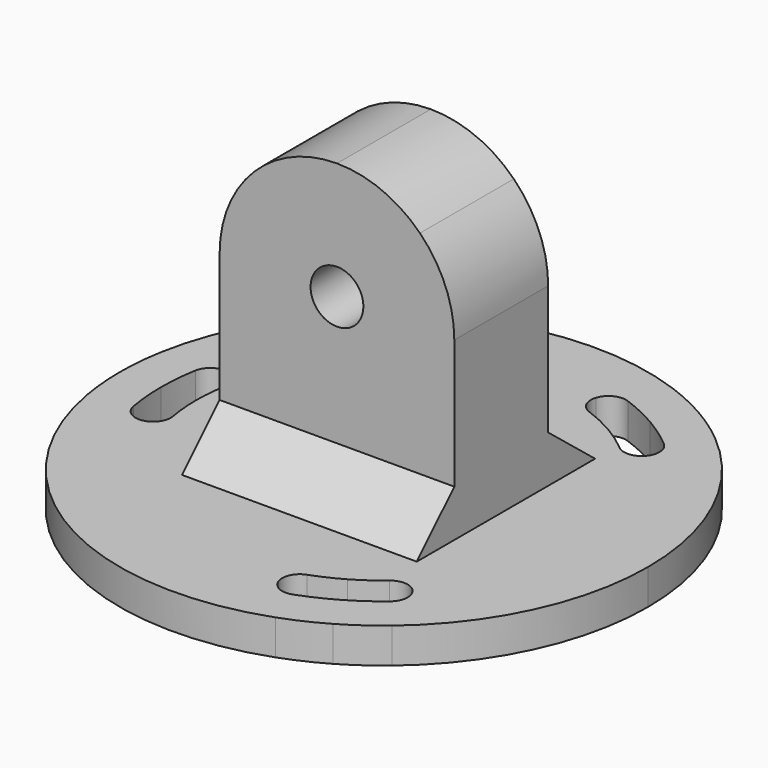
from build123d import *

# Parameters (mm, degrees)
F1_DEPTH = 6
F2_W     = 40
F2_H     = 20
F3_DEPTH = 50
F5_DEPTH = 40
F7_DEPTH = 30
F8_DEPTH = 30


# Not quite as in the source:
# - ends of sketch curves that miss each other by under 0.0002 mm in the source are joined


with BuildPart() as f1:
    # F0 (on Top) → F1 (new body)
    with BuildSketch(Plane.XY):
        with BuildLine():
            ThreePointArc((28.9254424359, -34.4719999404), (40.7838504166, -19.0178217783), (45, 0))
            ThreePointArc((45, 0), (40.7838504166, 19.0178217783), (28.9254424359, 34.4719999404))
            Line((28.9254424359, 34.4719999404), (24.4259291681, 29.1096888385))
            ThreePointArc((24.4259292345, 29.1096887828), (34.4396959257, 16.0594939069), (38, 0))
            ThreePointArc((38, 0), (34.4396959, -16.059493962), (24.4259291412, -29.1096888611))
            Line((24.4259291681, -29.1096888385), (28.9254424359, -34.4719999404))
        make_face()
        with BuildLine():
            ThreePointArc((22.5, -38.9711431703), (25.8109396358, -36.861841993), (28.9254424359, -34.4719999404))
            Line((28.9254424359, -34.4719999404), (24.4259291681, -29.1096888385))
            ThreePointArc((24.4259291412, -29.1096888611), (21.795904567, -31.127777693), (19, -32.9089653438))
            Line((19, -32.9089653438), (22.5, -38.9711431703))
        make_face()
        with BuildLine():
            ThreePointArc((15.3909064497, -42.2861679354), (19.0178217783, -40.7838504166), (22.5, -38.9711431703))
            Line((22.5, -38.9711431703), (19, -32.9089653438))
            ThreePointArc((19, -32.9089653438), (16.0594939837, -34.4396958899), (12.9967655243, -35.7083195615))
            Line((12.9967654464, -35.7083195899), (15.3909064497, -42.2861679354))
        make_face()
        with BuildLine():
            ThreePointArc((-44.3163488855, -7.814167995), (-22.5, -38.9711431703), (15.3909064497, -42.2861679354))
            Line((15.3909064497, -42.2861679354), (12.9967654464, -35.7083195899))
            ThreePointArc((12.9967655243, -35.7083195615), (-18.9999999457, -32.9089653752), (-37.4226946071, -6.5986307931))
            Line((-37.4226946145, -6.5986307513), (-44.3163488855, -7.814167995))
        make_face()
        with BuildLine():
            ThreePointArc((-37.4226946071, -6.5986307931), (-18.9999999457, -32.9089653752), (12.9967655243, -35.7083195615))
            ThreePointArc((12.9967655243, -35.7083195615), (10.6448654939, -35.5803659462), (9.1102432746, -33.7935418013))
            ThreePointArc((9.1102432746, -33.7935418013), (-17.5, -30.3108891325), (-33.8211873211, -9.0070687902))
            ThreePointArc((-33.8211873211, -9.0070687902), (-36.1359334802, -8.5714590704), (-37.4226946071, -6.5986307931))
        make_face()
        with BuildLine():
            ThreePointArc((-33.8211873211, -9.0070687902), (-17.5, -30.3108891325), (9.1102432746, -33.7935418013))
            ThreePointArc((9.1102432746, -33.7935418013), (9.2795808611, -31.5634020763), (10.9446447781, -30.0701637954))
            ThreePointArc((10.9446447781, -30.0701637954), (-15.9999999119, -27.712812972), (-31.5138480965, -5.5567416849))
            ThreePointArc((-31.5138480965, -5.5567416849), (-31.4796872612, -5.8162189899), (-31.4682713554, -6.0776862183))
            ThreePointArc((-31.4682713554, -6.0776862183), (-32.1293344064, -7.956349027), (-33.8211873211, -9.0070687902))
        make_face()
        with BuildLine():
            Line((10.9446445864, -30.0701638651), (0, 0))
            Line((0, 0), (-31.5138480964, -5.5567416853))
            ThreePointArc((-31.5138480964, -5.5567416853), (-15.9999999119, -27.712812972), (10.9446445864, -30.0701638651))
        make_face()
        with BuildLine():
            Line((-31.5138480964, -5.5567416853), (0, 0))
            Line((0, 0), (-32, 0))
            ThreePointArc((-32, 0), (-31.878230339, -2.7889837677), (-31.5138480965, -5.5567416849))
        make_face()
        with BuildLine():
            Line((-32, 0), (0, 0))
            Line((0, 0), (-31.5138480964, 5.5567416853))
            ThreePointArc((-31.5138480966, 5.5567416843), (-31.878230339, 2.7889837674), (-32, 0))
        make_face()
        with BuildLine():
            ThreePointArc((-45, 0), (-44.8287614141, -3.9220084236), (-44.3163488855, -7.814167995))
            Line((-44.3163488855, -7.814167995), (-37.4226946145, -6.5986307513))
            ThreePointArc((-37.4226946071, -6.5986307931), (-37.8553985256, -3.3119182456), (-38, 0))
            Line((-38, 0), (-45, 0))
        make_face()
        with BuildLine():
            Line((-37.4226946145, 6.5986307513), (-44.3163488855, 7.814167995))
            ThreePointArc((-44.3163488855, 7.814167995), (-44.8287614141, 3.9220084236), (-45, 0))
            Line((-45, 0), (-38, 0))
            ThreePointArc((-38, 0), (-37.8553985261, 3.3119182405), (-37.4226946089, 6.5986307831))
        make_face()
        with BuildLine():
            Line((12.9967654464, 35.7083195899), (15.3909064497, 42.2861679354))
            ThreePointArc((15.3909064497, 42.2861679354), (-22.5, 38.9711431703), (-44.3163488855, 7.814167995))
            Line((-44.3163488855, 7.814167995), (-37.4226946145, 6.5986307513))
            ThreePointArc((-37.4226946089, 6.5986307831), (-18.9999999501, 32.9089653726), (12.9967655243, 35.7083195615))
        make_face()
        with BuildLine():
            ThreePointArc((9.1102432746, 33.7935418013), (10.6448654939, 35.5803659462), (12.9967655243, 35.7083195615))
            ThreePointArc((12.9967655243, 35.7083195615), (-18.9999999501, 32.9089653726), (-37.4226946089, 6.5986307831))
            ThreePointArc((-37.4226946089, 6.5986307831), (-36.1359334844, 8.5714590676), (-33.8211873211, 9.0070687902))
            ThreePointArc((-33.8211873211, 9.0070687902), (-17.5, 30.3108891325), (9.1102432746, 33.7935418013))
        make_face()
        with BuildLine():
            Line((-31.5138480964, 5.5567416853), (0, 0))
            Line((0, 0), (10.9446445864, 30.0701638651))
            ThreePointArc((10.9446445864, 30.0701638651), (-15.9999999047, 27.7128129761), (-31.5138480964, 5.5567416853))
        make_face()
        with BuildLine():
            ThreePointArc((10.9446447943, 30.0701637895), (9.2795808649, 31.5634020686), (9.1102432746, 33.7935418013))
            ThreePointArc((9.1102432746, 33.7935418013), (-17.5, 30.3108891325), (-33.8211873211, 9.0070687902))
            ThreePointArc((-33.8211873211, 9.0070687902), (-32.1293344064, 7.956349027), (-31.4682713554, 6.0776862183))
            ThreePointArc((-31.4682713554, 6.0776862183), (-31.4796872612, 5.8162189895), (-31.5138480966, 5.5567416843))
            ThreePointArc((-31.5138480966, 5.5567416843), (-15.9999999047, 27.7128129761), (10.9446447943, 30.0701637895))
        make_face()
        with BuildLine():
            Line((19, 32.9089653438), (22.5, 38.9711431703))
            ThreePointArc((22.5, 38.9711431703), (19.0178217783, 40.7838504166), (15.3909064497, 42.2861679354))
            Line((15.3909064497, 42.2861679354), (12.9967654464, 35.7083195899))
            ThreePointArc((12.9967655243, 35.7083195615), (16.0594939837, 34.4396958899), (19, 32.9089653438))
        make_face()
        with BuildLine():
            Line((24.4259291681, 29.1096888385), (28.9254424359, 34.4719999404))
            ThreePointArc((28.9254424359, 34.4719999404), (25.8109396358, 36.861841993), (22.5, 38.9711431703))
            Line((22.5, 38.9711431703), (19, 32.9089653438))
            ThreePointArc((19, 32.9089653438), (21.7959046168, 31.1277776581), (24.4259292345, 29.1096887828))
        make_face()
        with BuildLine():
            Line((0, 0), (20.56920351, 24.5134221798))
            ThreePointArc((20.5692034907, 24.5134221959), (18.354445953, 26.2128654244), (16, 27.7128129211))
            Line((16, 27.7128129211), (0, 0))
        make_face()
        with BuildLine():
            Line((0, 0), (16, 27.7128129211))
            ThreePointArc((16, 27.7128129211), (13.523784476, 29.0018491384), (10.9446447943, 30.0701637895))
            Line((10.9446447943, 30.0701637895), (0, 0))
        make_face()
        with BuildLine():
            ThreePointArc((32, 0), (29.0018491799, 13.5237843871), (20.5692034907, 24.5134221959))
            Line((20.56920351, 24.5134221798), (0, 0))
            Line((0, 0), (20.56920351, -24.5134221798))
            ThreePointArc((20.5692034979, -24.5134221899), (29.0018491818, -13.5237843828), (32, 0))
        make_face()
        with BuildLine():
            ThreePointArc((16, -27.7128129211), (18.3544459568, -26.2128654218), (20.5692034979, -24.5134221899))
            Line((20.56920351, -24.5134221798), (0, 0))
            Line((0, 0), (16, -27.7128129211))
        make_face()
        with BuildLine():
            Line((16, -27.7128129211), (0, 0))
            Line((0, 0), (10.9446445864, -30.0701638651))
            ThreePointArc((10.9446445864, -30.0701638651), (13.5237844681, -29.0018491421), (16, -27.7128129211))
        make_face()
        with BuildLine():
            ThreePointArc((35, 0), (32.3255552282, 13.4185870786), (24.7109440465, 24.7864730111))
            ThreePointArc((24.7109440465, 24.7864730111), (22.6949176866, 23.8180538062), (20.5692034907, 24.5134221959))
            ThreePointArc((20.5692034907, 24.5134221959), (29.0018491799, 13.5237843871), (32, 0))
            ThreePointArc((32, 0), (29.0018491818, -13.5237843828), (20.5692034979, -24.5134221899))
            ThreePointArc((20.5692034979, -24.5134221899), (22.6949176913, -23.8180538065), (24.7109440465, -24.7864730111))
            ThreePointArc((24.7109440465, -24.7864730111), (32.3255552282, -13.4185870786), (35, 0))
        make_face()
        with BuildLine():
            ThreePointArc((38, 0), (34.4396959257, 16.0594939069), (24.4259292345, 29.1096887828))
            ThreePointArc((24.4259292345, 29.1096887828), (25.2164897185, 28.0794102551), (25.497566339, 26.8115555092))
            ThreePointArc((25.497566339, 26.8115555092), (25.294004531, 25.7253080978), (24.7109440465, 24.7864730111))
            ThreePointArc((24.7109440465, 24.7864730111), (32.3255552282, 13.4185870786), (35, 0))
            ThreePointArc((35, 0), (32.3255552282, -13.4185870786), (24.7109440465, -24.7864730111))
            ThreePointArc((24.7109440465, -24.7864730111), (25.294004531, -25.7253080978), (25.497566339, -26.8115555092))
            ThreePointArc((25.497566339, -26.8115555092), (25.2164896927, -28.0794103103), (24.4259291412, -29.1096888611))
            ThreePointArc((24.4259291412, -29.1096888611), (34.4396959, -16.059493962), (38, 0))
        make_face()
    extrude(amount=F1_DEPTH)

    # F2 (on face) → F3 (join)
    with BuildSketch(Plane.XY.offset(6)):
        Rectangle(F2_W, F2_H)
    extrude(amount=F3_DEPTH)

    # F4 (on face) → F5 (join)
    with BuildSketch(Plane(origin=(-20, 0, 0), x_dir=(0, -1, 0), z_dir=(-1, 0, 0))):
        Polygon((10, 14), (10, 6), (18, 6), align=None)
        Polygon((-10, 14), (-20, 6), (-10, 6), align=None)
    extrude(amount=-F5_DEPTH)

    # F6 (on face) → F7 (cut)
    with BuildSketch(Plane.XZ.offset(10)):
        with BuildLine():
            Line((-14.1421356237, 50.1421356237), (-20, 56))
            Line((-20, 56), (-20, 36))
            ThreePointArc((-20, 36), (-18.4775906502, 43.6536686473), (-14.1421356237, 50.1421356237))
        make_face()
        with BuildLine():
            Line((1.654e-07, 56), (-20, 56))
            Line((-20, 56), (-14.1421356237, 50.1421356237))
            ThreePointArc((-14.1421356237, 50.1421356237), (-7.6536685709, 54.4775906819), (1.654e-07, 56))
        make_face()
        with BuildLine():
            Line((20, 56), (1.654e-07, 56))
            ThreePointArc((1.654e-07, 56), (7.6536687237, 54.4775906186), (14.1421356237, 50.1421356237))
            Line((14.1421356237, 50.1421356237), (20, 56))
        make_face()
        with BuildLine():
            Line((20, 56), (14.1421356237, 50.1421356237))
            ThreePointArc((14.1421356237, 50.1421356237), (18.4775906502, 43.6536686473), (20, 36))
            Line((20, 36), (20, 56))
        make_face()
    extrude(amount=-F7_DEPTH, mode=Mode.SUBTRACT)

    # F6 (on face) → F8 (cut)
    with BuildSketch(Plane.XZ.offset(10)):
        with BuildLine():
            Line((0, 36), (-3.1819805153, 39.1819805153))
            ThreePointArc((-3.1819805153, 39.1819805153), (-1.7220754456, 31.8425421037), (4.5, 36))
            ThreePointArc((4.5, 36), (4.1574578963, 37.7220754456), (3.1819805153, 39.1819805153))
            Line((3.1819805153, 39.1819805153), (0, 36))
        make_face()
        with BuildLine():
            ThreePointArc((3.1819805153, 39.1819805153), (0, 40.5), (-3.1819805153, 39.1819805153))
            Line((-3.1819805153, 39.1819805153), (0, 36))
            Line((0, 36), (3.1819805153, 39.1819805153))
        make_face()
    extrude(amount=-F8_DEPTH, mode=Mode.SUBTRACT)


solid = f1.part
